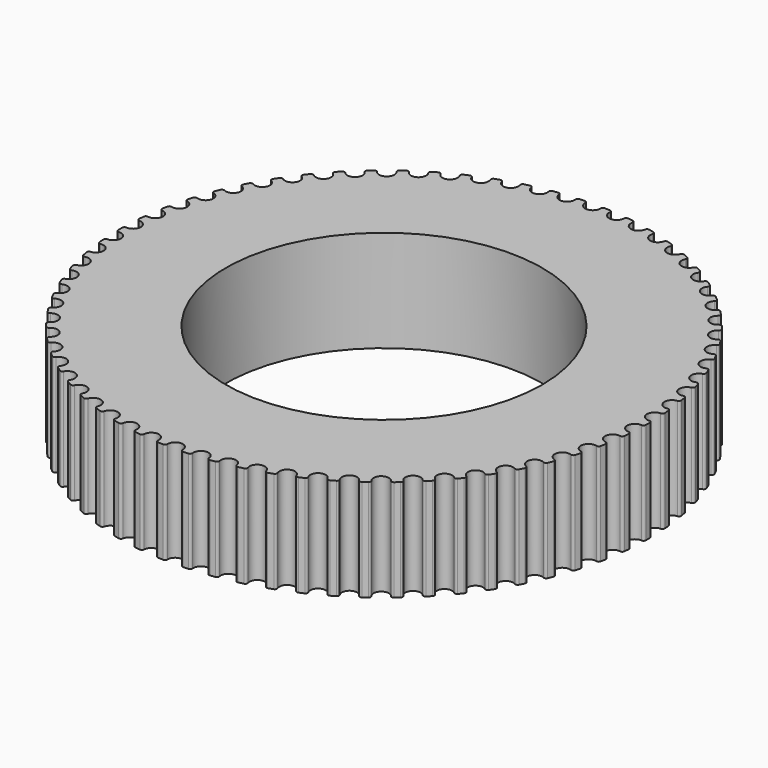
from build123d import *

# Parameters (mm, degrees)
F2_R            = 51.9486312803
F3_DEPTH        = 20
F5_DEPTH        = 20
F5_COPIES_COUNT = 66
F7_R            = 31.15
F8_DEPTH        = 25


# Not quite as in the source:
# - a feature of the source that left no trace in its solid (it failed there, or was rolled back) is left out
# - a pattern or mirror of a feature is missing from the dataset's text; its kind, count and spacing are read off the source's solid


with BuildPart() as f3:
    # F2 (on Top) → F3 (new body)
    with BuildSketch(Plane.XY):
        Circle(F2_R)
    extrude(amount=F3_DEPTH)

    # F4 (on face) → F5 (cut, through all)
    with BuildSketch(Plane.XY.offset(20)):
        with BuildLine():
            ThreePointArc((-1.9656559066, 51.9114292691), (-1.6304848293, 51.7800038488), (-1.4989450786, 51.4448776246))
            ThreePointArc((-1.4989450786, 51.4448776246), (0, 49.8886312803), (1.4989450786, 51.4448776246))
            ThreePointArc((1.4989450786, 51.4448776246), (1.6304848293, 51.7800038488), (1.9656559066, 51.9114292691))
            ThreePointArc((1.9656559066, 51.9114292691), (0, 51.9486312803), (-1.9656559066, 51.9114292691))
        make_face()
    f5 = extrude(amount=-F5_DEPTH, mode=Mode.SUBTRACT)

    # F5_copies: F5 ×66 about axis
    f5_copies_axis = Axis((0, 0, 0), (0, 0, 1))
    for i in range(1, F5_COPIES_COUNT):
        add(f5.rotate(f5_copies_axis, i * 360 / F5_COPIES_COUNT), mode=Mode.SUBTRACT)

    # F7 (on face) → F8 (cut)
    with BuildSketch(Plane(origin=(0, 0, 0), x_dir=(1, 0, 0), z_dir=(0, 0, -1))):
        Circle(F7_R)
    extrude(amount=-F8_DEPTH, mode=Mode.SUBTRACT)


solid = f3.part
